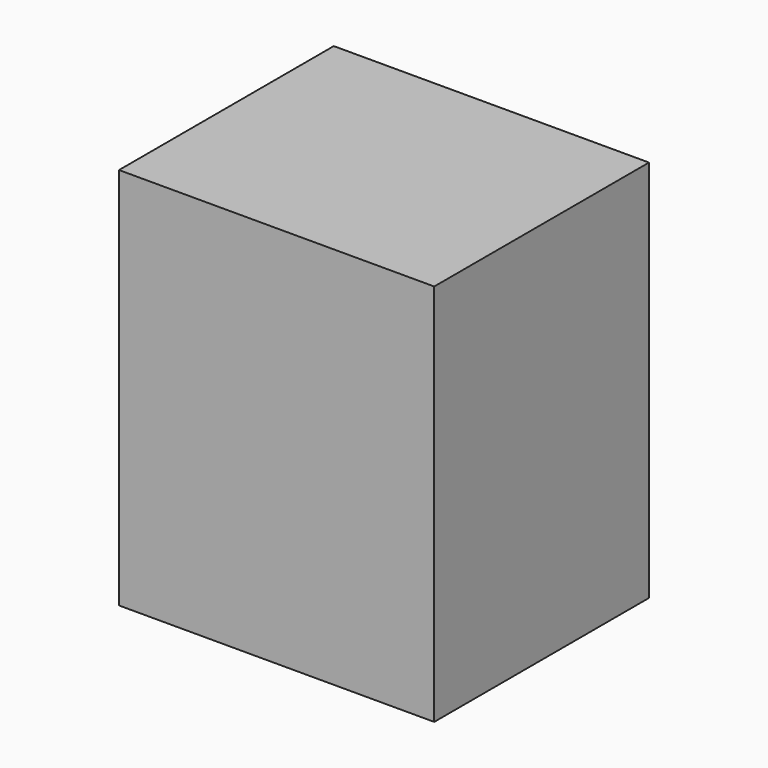
from build123d import *

# Parameters (mm, degrees)
F0_W     = 29.8250038177
F0_H     = 36.2700223923
F1_DEPTH = 25.4


# Not quite as in the source:
# - a feature names something its author has since deleted; it is built from what else it names


with BuildPart() as f1:
    # F0 (on Front) → F1 (new body)
    with BuildSketch(Plane.XZ):
        with Locations((-14.9125019088, -18.1350111961)):
            Rectangle(F0_W, F0_H)
    extrude(amount=-F1_DEPTH)


solid = f1.part
